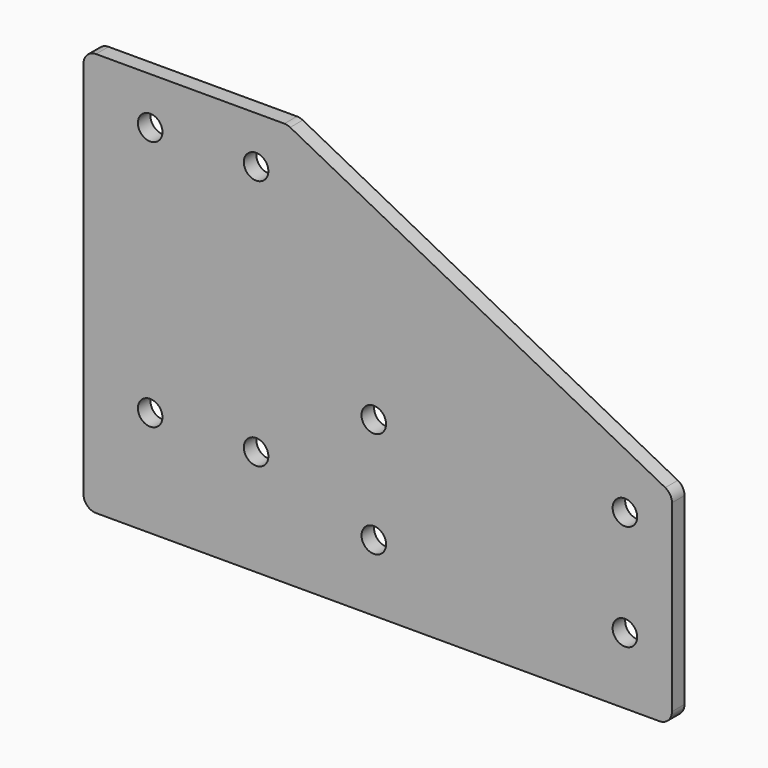
from build123d import *

# Parameters (mm, degrees)
F0_R     = 4.9657
F1_DEPTH = 6.35
F2_R     = 5.08


# Not quite as in the source:
# - a feature names something its author has since deleted; it is built from what else it names


with BuildPart() as f1:
    # F0 (on Front) → F1 (new body)
    with BuildSketch(Plane.XZ):
        Polygon((-96.7471700311, 0.2120000629), (141.3778299689, 0.2120000629), (141.3778299689, 82.7620000629), (-14.1971700311, 163.7245000629), (-96.7471700311, 163.7245000629), (-96.7471700311, 144.6745000629), align=None)
        with Locations((20.7278299689, 27.1995000629)):
            Circle(F0_R, mode=Mode.SUBTRACT)
        with Locations((-69.7596700311, 43.0745000629)):
            Circle(F0_R, mode=Mode.SUBTRACT)
        with Locations((-26.8971700311, 43.0745000629)):
            Circle(F0_R, mode=Mode.SUBTRACT)
        with Locations((20.7278299689, 70.0620000629)):
            Circle(F0_R, mode=Mode.SUBTRACT)
        with Locations((122.3278299689, 27.1995000629)):
            Circle(F0_R, mode=Mode.SUBTRACT)
        with Locations((122.3278299689, 70.0620000629)):
            Circle(F0_R, mode=Mode.SUBTRACT)
        with BuildLine():
            ThreePointArc((-64.7939700311, 144.6745000629), (-69.7596700311, 139.7088000629), (-74.7253700311, 144.6745000629))
            ThreePointArc((-74.7253700311, 144.6745000629), (-69.7596700311, 149.6402000629), (-64.7939700311, 144.6745000629))
        make_face(mode=Mode.SUBTRACT)
        with Locations((-26.8971700311, 144.6745000629)):
            Circle(F0_R, mode=Mode.SUBTRACT)
    extrude(amount=F1_DEPTH)

    # F2
    f2_edges = [f1.edges().sort_by_distance(p)[0] for p in [
        (-96.74717, -3.175, 0.212),
        (-96.74717, -3.175, 163.7245),
        (-14.19717, -3.175, 163.7245),
        (141.37783, -3.175, 82.762),
        (141.37783, -3.175, 0.212),
    ]]
    fillet(f2_edges, radius=F2_R)


solid = f1.part
